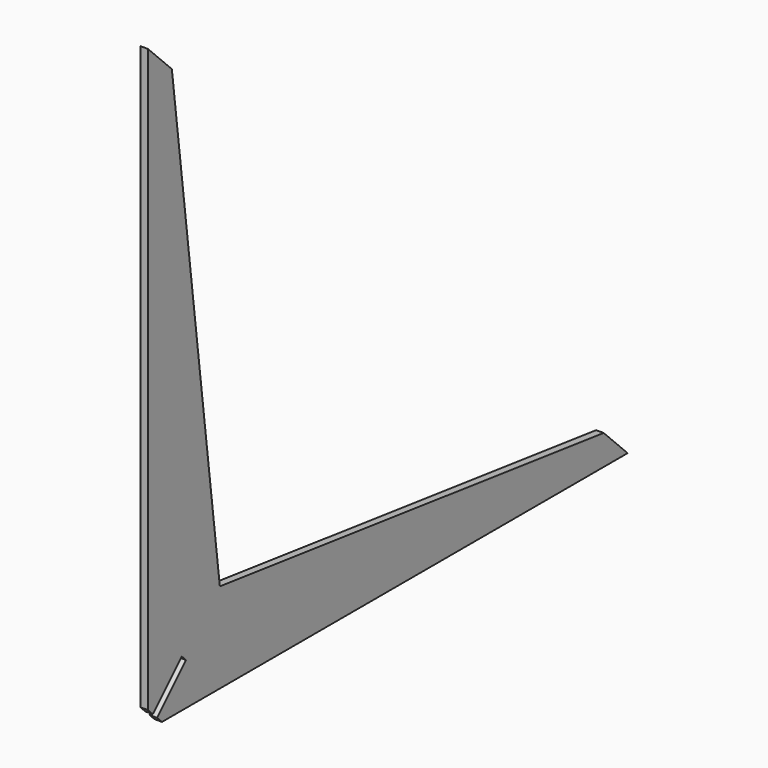
from build123d import *

# Parameters (mm, degrees)
F1_DEPTH = 12.7
F3_DEPTH = 12.701
F5_DEPTH = 12.701


# Not quite as in the source:
# - a length typed as a fraction of an inch, garbled in the dataset ("3 / 203.2 mm" for 3/8 in), is restored


with BuildPart() as f1:
    # F0 (on Right) → F1 (new body)
    with BuildSketch(Plane.YZ):
        Polygon((-313.2666666667, 601.1333333333), (-364.0666666667, 651.9333333333), (-364.0666666667, -364.0666666667), (651.9333333333, -364.0666666667), (601.1333333333, -313.2666666667), (-211.6666666667, -211.6666666667), align=None)
    extrude(amount=F1_DEPTH)

    # F2 (on face) → F3 (cut, through all)
    with BuildSketch(Plane.YZ.offset(12.7)):
        Polygon((-283.3765386061, -292.3567947272), (-287.8666666667, -287.8666666667), (-292.3567947272, -283.3765386061), (-364.0666666667, -355.0864105456), (-364.0666666667, -364.0666666667), (-355.0864105456, -364.0666666667), align=None)
    extrude(amount=-F3_DEPTH, mode=Mode.SUBTRACT)

    # F4 (on face) → F5 (cut, through all)
    with BuildSketch(Plane.YZ.offset(12.7)):
        Polygon((-334.1487050056, -364.0666666667), (-364.0666666667, -334.1487050056), (-364.0666666667, -355.0864105456), (-355.0864105456, -364.0666666667), align=None)
    extrude(amount=-F5_DEPTH, mode=Mode.SUBTRACT)


solid = f1.part
